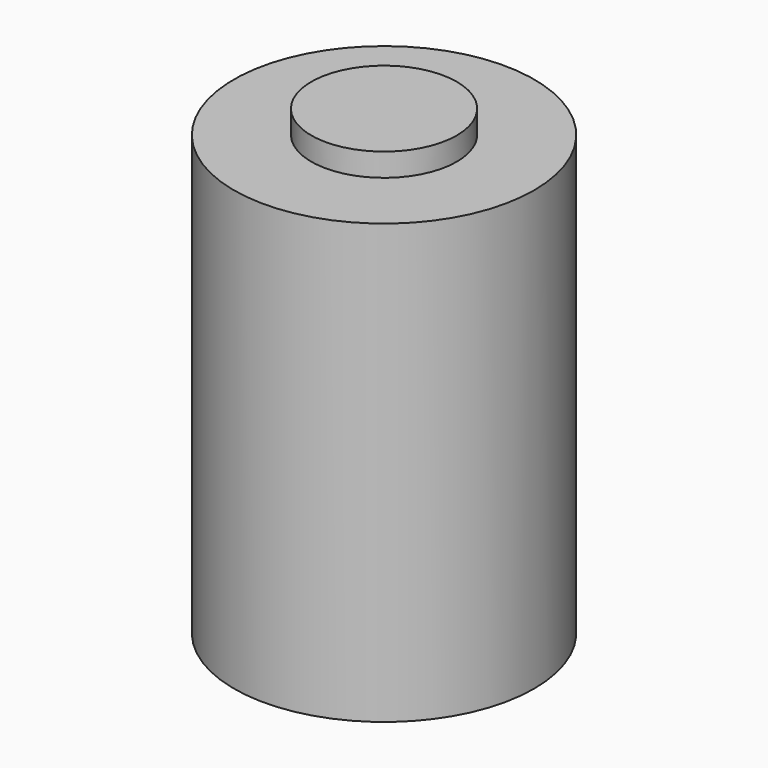
from build123d import *

# Parameters (mm, degrees)
F0_R     = 3.25
F0_R_2   = 1.575
F1_DEPTH = 9.5
F2_DEPTH = 10


# Not quite as in the source:
# - a feature of the source that left no trace in its solid (it failed there, or was rolled back) is left out


with BuildPart() as f1:
    # F0 (on Top) → F1 (new body)
    with BuildSketch(Plane.XY):
        Circle(F0_R)
        Circle(F0_R_2, mode=Mode.SUBTRACT)
    extrude(amount=F1_DEPTH)

    # F0 (on Top) → F2 (join)
    with BuildSketch(Plane.XY):
        Circle(F0_R_2)
    extrude(amount=F2_DEPTH)


solid = f1.part
